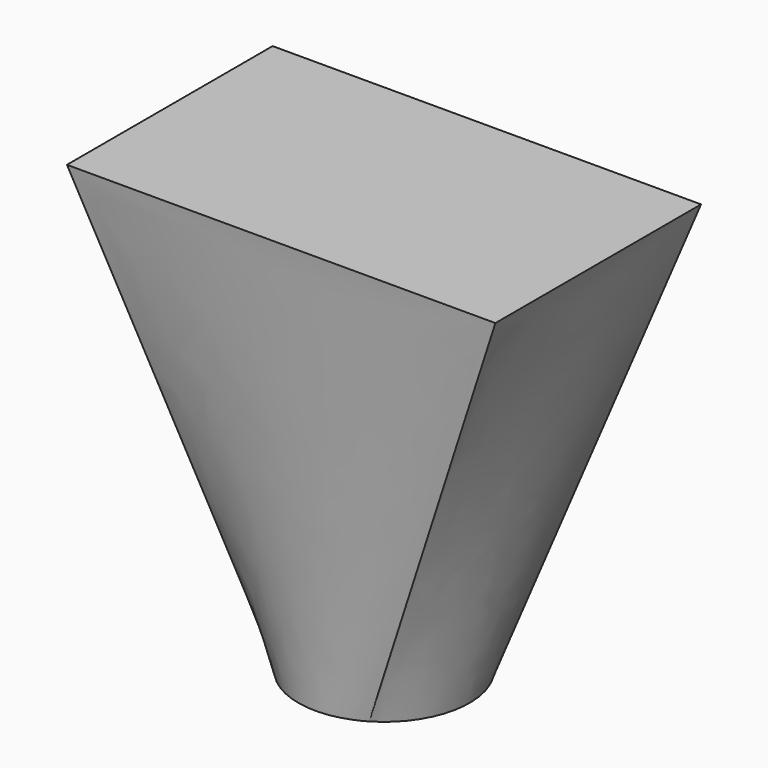
from build123d import *

# Parameters (mm, degrees)
F2_W = 127
F2_H = 76.2


# Not quite as in the source:
# - the arcs of a loft's sections are written as splines that run evenly, so that the points pair up as in the source's solid


with BuildPart() as f3:
    # F0 (on Top) → F3 section 0
    with BuildSketch(Plane.XY):
        with BuildLine():
            add(Edge.make_bspline(
                [(21.7803203131, 13.0681921879), (20.9250091345, 14.4937108189), (19.9293212464, 15.8349554859), (17.6953582406, 18.2974849998), (16.457138362, 19.4187089559), (13.7856846531, 21.3980970935), (12.3525168797, 22.2562123309), (9.3462349355, 23.6763923162), (7.773195101, 24.2384219474), (4.5476146508, 25.04481706), (2.8951537939, 25.2891626016), (-0.4257679146, 25.4507835294), (-2.0941466499, 25.3680549193), (-5.3827884578, 24.8786906608), (-7.0029702123, 24.472067113), (-10.1329514593, 23.3505236623), (-11.6426735568, 22.6356314917), (-13.0681921879, 21.7803203131)],
                knots=[0, 0, 0, 0, 0.125, 0.125, 0.25, 0.25, 0.375, 0.375, 0.5, 0.5, 0.625, 0.625, 0.75, 0.75, 0.875, 0.875, 1, 1, 1, 1], degree=3))
            add(Edge.make_bspline(
                [(-13.0681921879, 21.7803203131), (-14.4937108189, 20.9250091345), (-15.8349554859, 19.9293212464), (-18.2974849998, 17.6953582406), (-19.4187089559, 16.457138362), (-21.3980970935, 13.7856846531), (-22.2562123309, 12.3525168797), (-23.6763923162, 9.3462349355), (-24.2384219474, 7.773195101), (-25.04481706, 4.5476146508), (-25.2891626016, 2.8951537939), (-25.4507835294, -0.4257679146), (-25.3680549193, -2.0941466499), (-24.8786906608, -5.3827884578), (-24.472067113, -7.0029702123), (-23.3505236623, -10.1329514593), (-22.6356314917, -11.6426735568), (-21.7803203131, -13.0681921879)],
                knots=[0, 0, 0, 0, 0.125, 0.125, 0.25, 0.25, 0.375, 0.375, 0.5, 0.5, 0.625, 0.625, 0.75, 0.75, 0.875, 0.875, 1, 1, 1, 1], degree=3))
            add(Edge.make_bspline(
                [(-21.7803203131, -13.0681921879), (-20.9250091345, -14.4937108189), (-19.9293212464, -15.8349554859), (-17.6953582406, -18.2974849998), (-16.457138362, -19.4187089559), (-13.7856846531, -21.3980970935), (-12.3525168797, -22.2562123309), (-9.3462349355, -23.6763923162), (-7.773195101, -24.2384219474), (-4.5476146508, -25.04481706), (-2.8951537939, -25.2891626016), (0.4257679146, -25.4507835294), (2.0941466499, -25.3680549193), (5.3827884578, -24.8786906608), (7.0029702123, -24.472067113), (10.1329514593, -23.3505236623), (11.6426735568, -22.6356314917), (13.0681921879, -21.7803203131)],
                knots=[0, 0, 0, 0, 0.125, 0.125, 0.25, 0.25, 0.375, 0.375, 0.5, 0.5, 0.625, 0.625, 0.75, 0.75, 0.875, 0.875, 1, 1, 1, 1], degree=3))
            add(Edge.make_bspline(
                [(13.0681921879, -21.7803203131), (14.4937108189, -20.9250091345), (15.8349554859, -19.9293212464), (18.2974849998, -17.6953582406), (19.4187089559, -16.457138362), (21.3980970935, -13.7856846531), (22.2562123309, -12.3525168797), (23.6763923162, -9.3462349355), (24.2384219474, -7.773195101), (25.04481706, -4.5476146508), (25.2891626016, -2.8951537939), (25.4507835294, 0.4257679146), (25.3680549193, 2.0941466499), (24.8786906608, 5.3827884578), (24.472067113, 7.0029702123), (23.3505236623, 10.1329514593), (22.6356314917, 11.6426735568), (21.7803203131, 13.0681921879)],
                knots=[0, 0, 0, 0, 0.125, 0.125, 0.25, 0.25, 0.375, 0.375, 0.5, 0.5, 0.625, 0.625, 0.75, 0.75, 0.875, 0.875, 1, 1, 1, 1], degree=3))
        make_face()
    # F2 (on offset) → F3 section 1
    with BuildSketch(Plane.XY.offset(127)):
        Rectangle(F2_W, F2_H)
    loft(ruled=True)


solid = f3.part
